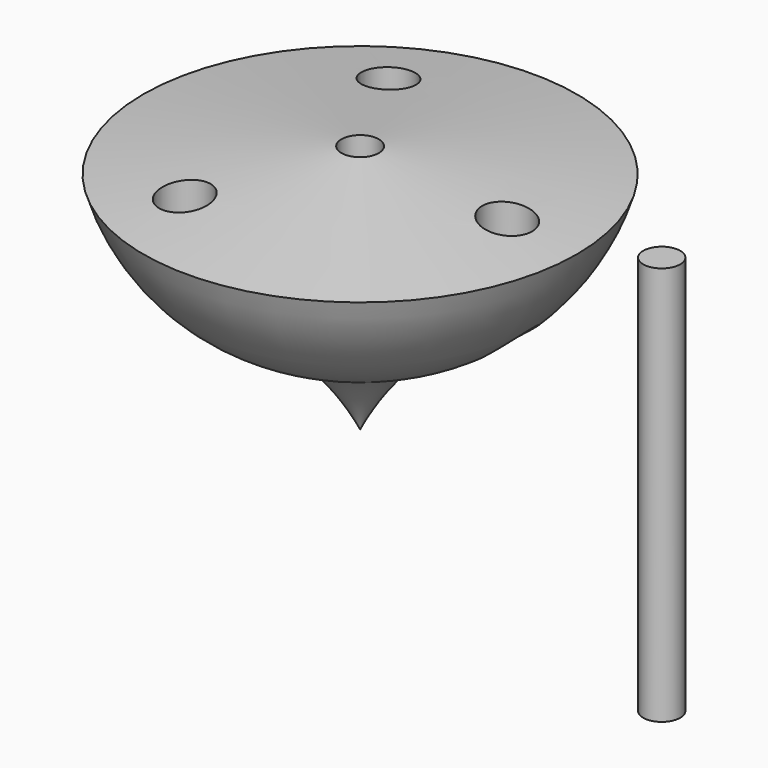
from build123d import *

# Parameters (mm, degrees)
F3_D          = 6.35
F4_R          = 2.3495
F5_DEPTH      = 31.75
F5_DEPTH_BACK = 19.05


# Not quite as in the source:
# - a feature names something its author has since deleted; it is built from what else it names


with BuildPart() as f1:
    # F0 (on Front) → F1 (revolve)
    with BuildSketch(Plane.XZ):
        with BuildLine():
            Line((0, 19.05), (0, 0))
            ThreePointArc((0, 0), (3.6250012472, 5.7505099882), (8.3881448954, 10.6004029512))
            ThreePointArc((8.3881448954, 10.6004029512), (20.4323715587, 16.9914499437), (27.5851080685, 28.5995177414))
            Line((27.5851080685, 28.5995177414), (2.38125, 31.75))
            Line((2.38125, 31.75), (2.38125, 19.05))
            Line((2.38125, 19.05), (0, 19.05))
        make_face()
    revolve(axis=Axis((0, 0, 9.525), (0, 0, -1)))

    # F3 (through all)
    with Locations(Plane(origin=(0, 0, 0), x_dir=(1, 0, 0), z_dir=(0, 0, -1))):
        with Locations((18.7120120972, 0), (-9.3560060486, -16.2050778321), (-9.3560060486, 16.2050778321)):
            Hole(F3_D / 2)


with BuildPart() as f5:
    # F4 (on Top) → F5 (new body, two sides)
    with BuildSketch(Plane.XY) as f5_sk:
        with Locations((38.3784368877, 0)):
            Circle(F4_R)
    extrude(amount=F5_DEPTH)
    extrude(f5_sk.sketch, amount=-F5_DEPTH_BACK)


solid = Compound([f1.part, f5.part])
